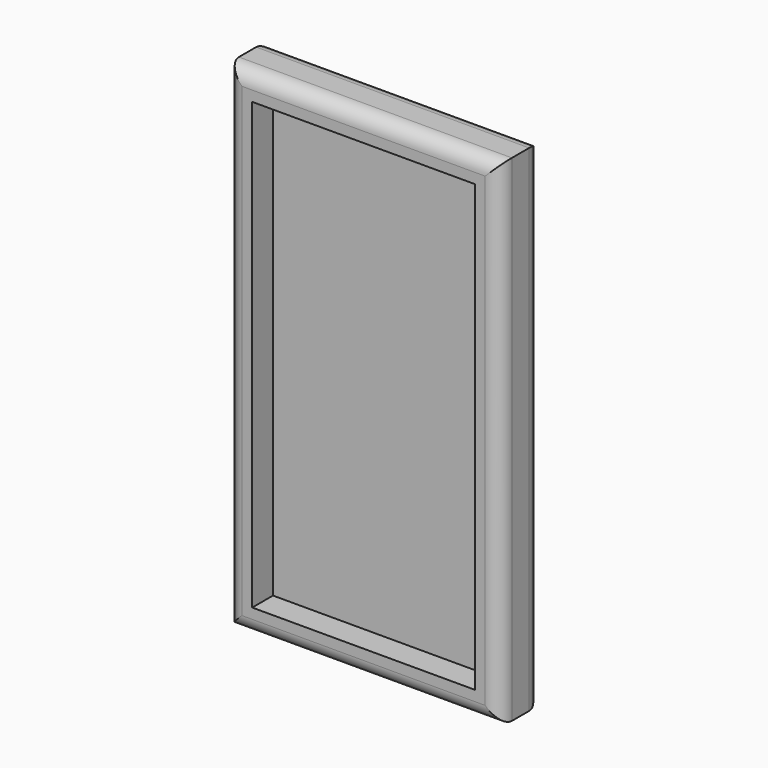
from build123d import *

# Parameters (mm, degrees)
F0_W        = 76.2
F0_H        = 152.4
F1_DEPTH    = 8.89
F2_T        = 8.636
F3_T1_DEPTH = 118.872
F3_T3_DEPTH = 195.072


# Not quite as in the source:
# - a fillet or chamfer that OpenCascade refuses, or shapes differently, is made with other operations: its cross-section is extruded or revolved along the edge and cut away or added


with BuildPart() as f1:
    # F0 (on Front) → F1 (new body)
    with BuildSketch(Plane.XZ):
        with Locations((1.7131138593, 3.2272135141)):
            Rectangle(F0_W, F0_H)
    extrude(amount=F1_DEPTH)

    # F2
    f2_openings = [f1.faces().sort_by_distance(p)[0] for p in [
        (1.713114, -8.89, 3.227214),
    ]]
    offset(amount=F2_T, openings=f2_openings, kind=Kind.INTERSECTION)

    # F3: fillet of radius 5.08 on 8 edges, made by hand

    # F3_s2 → F3_t1 (cut)
    with BuildSketch(Plane.YZ.offset(-57.7228861407)):
        with BuildLine():
            ThreePointArc((-8.89, -76.5287864859), (-7.4021024484, -80.1208889343), (-3.81, -81.6087864859))
            Line((-3.81, -81.6087864859), (-8.89, -81.6087864859))
            Line((-8.89, -81.6087864859), (-8.89, -76.5287864859))
        make_face()
        with BuildLine():
            ThreePointArc((-8.89, 82.9832135141), (-7.4021024484, 86.5753159626), (-3.81, 88.0632135141))
            Line((-3.81, 88.0632135141), (-8.89, 88.0632135141))
            Line((-8.89, 88.0632135141), (-8.89, 82.9832135141))
        make_face()
        with BuildLine():
            ThreePointArc((3.556, 88.0632135141), (7.1481024484, 86.5753159626), (8.636, 82.9832135141))
            Line((8.636, 82.9832135141), (8.636, 88.0632135141))
            Line((8.636, 88.0632135141), (3.556, 88.0632135141))
        make_face()
        with BuildLine():
            ThreePointArc((3.556, -81.6087864859), (7.1481024484, -80.1208889343), (8.636, -76.5287864859))
            Line((8.636, -76.5287864859), (8.636, -81.6087864859))
            Line((8.636, -81.6087864859), (3.556, -81.6087864859))
        make_face()
    extrude(amount=F3_T1_DEPTH, mode=Mode.SUBTRACT)

    # F3_s4 → F3_t3 (cut)
    with BuildSketch(Plane.XY.offset(-94.3087864859)):
        with BuildLine():
            ThreePointArc((43.3691138593, -8.89), (46.9612163077, -7.4021024484), (48.4491138593, -3.81))
            Line((48.4491138593, -3.81), (48.4491138593, -8.89))
            Line((48.4491138593, -8.89), (43.3691138593, -8.89))
        make_face()
        with BuildLine():
            ThreePointArc((-39.9428861407, -8.89), (-43.5349885891, -7.4021024484), (-45.0228861407, -3.81))
            Line((-45.0228861407, -3.81), (-45.0228861407, -8.89))
            Line((-45.0228861407, -8.89), (-39.9428861407, -8.89))
        make_face()
        with BuildLine():
            ThreePointArc((-45.0228861407, 3.556), (-43.5349885891, 7.1481024484), (-39.9428861407, 8.636))
            Line((-39.9428861407, 8.636), (-45.0228861407, 8.636))
            Line((-45.0228861407, 8.636), (-45.0228861407, 3.556))
        make_face()
        with BuildLine():
            ThreePointArc((48.4491138593, 3.556), (46.9612163077, 7.1481024484), (43.3691138593, 8.636))
            Line((43.3691138593, 8.636), (48.4491138593, 8.636))
            Line((48.4491138593, 8.636), (48.4491138593, 3.556))
        make_face()
    extrude(amount=F3_T3_DEPTH, mode=Mode.SUBTRACT)


solid = f1.part
